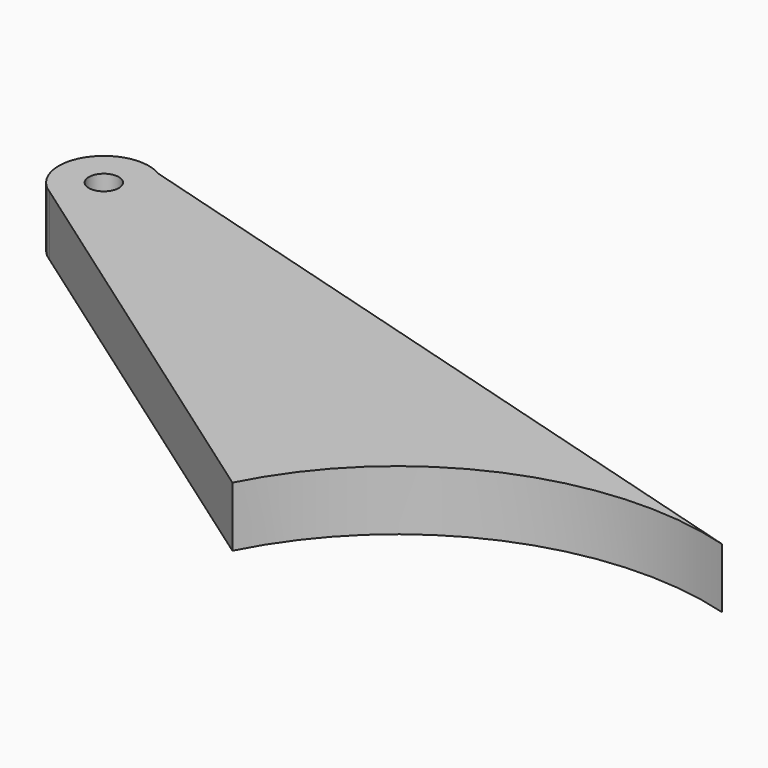
from build123d import *

# Parameters (mm, degrees)
F0_R     = 0.75
F1_DEPTH = 3


# Not quite as in the source:
# - a feature names something its author has since deleted; it is built from what else it names


with BuildPart() as f1:
    # F0 (on Top) → F1 (new body)
    with BuildSketch(Plane.XY):
        with BuildLine():
            ThreePointArc((-13.8337529302, 6.9912287808), (-6.1730560637, 14.2177135586), (4.3373536701, 14.8807715909))
            Line((4.3373536701, 14.8807715909), (-32.4411373594, 25.6007347374))
            ThreePointArc((-32.4411373594, 25.6007347374), (-35.456761187, 24.972624675), (-35.0323544011, 21.9216595489))
            Line((-35.0323544011, 21.9216595489), (-34.7850043318, 21.747447911))
            Line((-34.7850043318, 21.747447911), (-13.8337529302, 6.9912287808))
        make_face()
        with Locations((-33.6130708456, 23.6740913242)):
            Circle(F0_R, mode=Mode.SUBTRACT)
    extrude(amount=F1_DEPTH)


solid = f1.part
